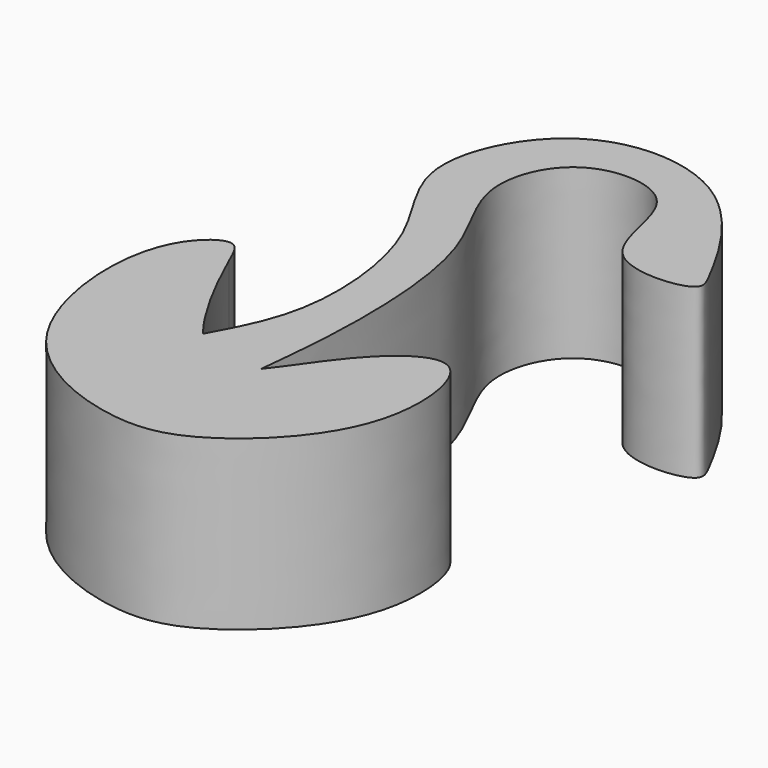
from build123d import *

# Parameters (mm, degrees)
F1_DEPTH = 12.7


# Not quite as in the source:
# - a feature of the source that left no trace in its solid (it failed there, or was rolled back) is left out


with BuildPart() as f1:
    # F0 (on Top) → F1 (new body)
    with BuildSketch(Plane.XY):
        with BuildLine():
            add(Edge.make_bspline(
                [(-12.9939224571, 6.646854803), (-12.0209842013, 4.444653204), (-10.2419200653, 0.7550026988), (-8.3734039217, -1.5674004098)],
                knots=[0, 0, 0, 0, 0.1008239216, 0.1008239216, 0.1008239216, 0.1008239216], degree=3))
            add(Edge.make_bspline(
                [(-2.8972320724, -2.9364430811), (-1.776177319, -1.5731363584), (0.7707430366, 2.7151758339), (6.5018929938, 6.1730497094), (8.2616317976, -4.5662684102), (0.3213481372, -12.577111166), (-6.0175770538, -13.8084879138), (-17.4512622323, -9.1891533031), (-18.9653411147, 5.5420981515), (-14.1400034064, 9.4349451722), (-13.4774376543, 7.7412695142), (-12.9939224571, 6.646854803)],
                knots=[0.2188999646, 0.2188999646, 0.2188999646, 0.2188999646, 0.3054765878, 0.3747524984, 0.4664373696, 0.573990642, 0.6550811044, 0.7634569353, 0.8832783199, 0.94989415, 1, 1, 1, 1], degree=3))
            add(Edge.make_bspline(
                [(-8.3734039217, -1.5674004098), (-7.0943249904, -3.1571843121), (-4.8343729552, -4.7808880912), (-3.53246646, -3.7089471078), (-2.8972320724, -2.9364430811)],
                knots=[0.1008239216, 0.1008239216, 0.1008239216, 0.1008239216, 0.1698421928, 0.2188999646, 0.2188999646, 0.2188999646, 0.2188999646], degree=3))
        make_face()
        with BuildLine():
            add(Edge.make_bspline(
                [(-8.3734039217, -1.5674004098), (-7.3043582316, 0.3830967726), (-4.9024380761, 4.7654524935), (-6.1430653348, 16.2348730997), (-12.6758917382, 23.0174740706), (-7.4792433532, 33.8377035792), (4.8274970419, 33.2079692165), (10.0745612008, 23.3085390875), (11.4394480919, 20.6824307654), (2.690343607, 20.0416706357), (3.7484964525, 29.7469283628), (-4.9894882783, 30.2995644972), (-7.803620131, 23.1321761316), (-2.7268516768, 16.8852917181), (-2.0428900587, 5.1729754673), (-2.6288507594, -0.3889663524), (-2.8972320724, -2.9364430811)],
                knots=[0, 0, 0, 0, 0.0683400172, 0.1535456026, 0.2295771238, 0.3082347453, 0.391106723, 0.4753014914, 0.5089882749, 0.570764487, 0.6405741543, 0.7041245781, 0.7672384461, 0.8383843918, 0.9259769314, 1, 1, 1, 1], degree=3))
            add(Edge.make_bspline(
                [(-8.3734039217, -1.5674004098), (-7.0943249904, -3.1571843121), (-4.8343729552, -4.7808880912), (-3.53246646, -3.7089471078), (-2.8972320724, -2.9364430811)],
                knots=[0.1008239216, 0.1008239216, 0.1008239216, 0.1008239216, 0.1698421928, 0.2188999646, 0.2188999646, 0.2188999646, 0.2188999646], degree=3))
        make_face()
    extrude(amount=F1_DEPTH)


solid = f1.part
